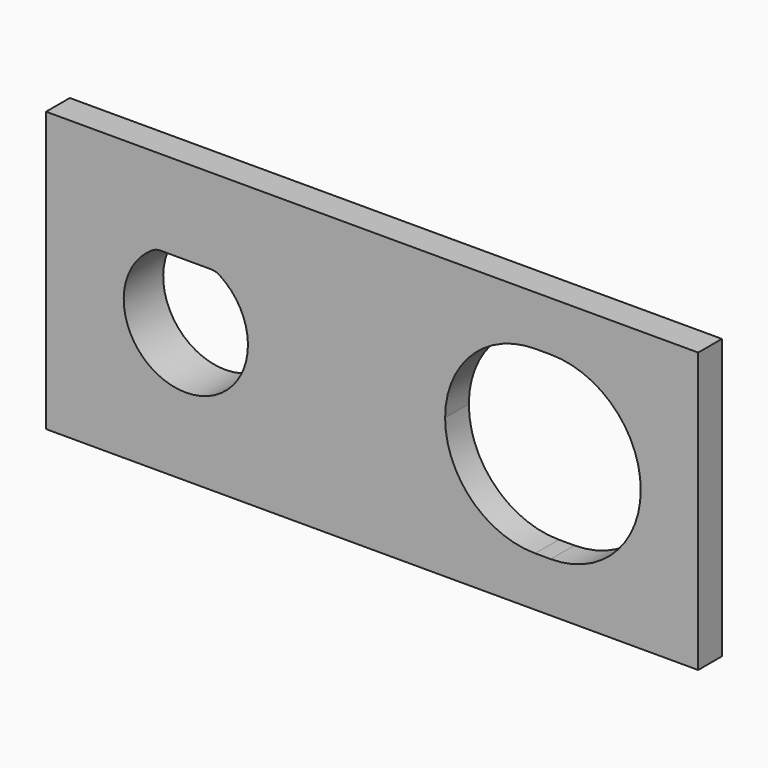
from build123d import *

# Parameters (mm, degrees)
F0_W     = 42
F0_H     = 18
F2_DEPTH = 1.91
F1_R     = 4.6
F3_DEPTH = 3.18
F4_SIZE  = 0.25


# Not quite as in the source:
# - a feature names something its author has since deleted; it is built from what else it names


with BuildPart() as f2:
    # F0 (on Front) → F2 (new body)
    with BuildSketch(Plane.XZ):
        with Locations((21, 9)):
            Rectangle(F0_W, F0_H)
        with BuildLine():
            ThreePointArc((11.1703455946, 12.36), (9, 5), (6.8296544054, 12.36))
            ThreePointArc((6.8296544054, 12.36), (7.0893980916, 12.4791663047), (7.372240804, 12.52))
            Line((7.372240804, 12.52), (10.627759196, 12.52))
            ThreePointArc((10.627759196, 12.52), (10.9106019084, 12.4791663047), (11.1703455946, 12.36))
        make_face(mode=Mode.SUBTRACT)
        with BuildLine():
            Line((32.5, 3.2), (31.5, 3.2))
            ThreePointArc((31.5, 3.2), (27.3987806691, 4.8987806691), (25.7, 9))
            ThreePointArc((25.7, 9), (27.3987806691, 13.1012193309), (31.5, 14.8))
            Line((31.5, 14.8), (32.5, 14.8))
            ThreePointArc((32.5, 14.8), (36.6012193309, 13.1012193309), (38.3, 9))
            ThreePointArc((38.3, 9), (36.6012193309, 4.8987806691), (32.5, 3.2))
        make_face(mode=Mode.SUBTRACT)
    extrude(amount=-F2_DEPTH)

    # F1 (on face) → F3 (join)
    with BuildSketch(Plane.XZ):
        with Locations((9, 9)):
            Circle(F1_R)
        with BuildLine():
            ThreePointArc((10.627759196, 12.52), (10.9106019084, 12.4791663047), (11.1703455946, 12.36))
            ThreePointArc((11.1703455946, 12.36), (9, 5), (6.8296544054, 12.36))
            ThreePointArc((6.8296544054, 12.36), (7.0893980916, 12.4791663047), (7.372240804, 12.52))
            Line((7.372240804, 12.52), (10.627759196, 12.52))
        make_face(mode=Mode.SUBTRACT)
    extrude(amount=-F3_DEPTH)

    # F4
    f4_edges = [f2.edges().sort_by_distance(p)[0] for p in [
        (4.4, 3.18, 9),
    ]]
    chamfer(f4_edges, length=F4_SIZE)


solid = f2.part
